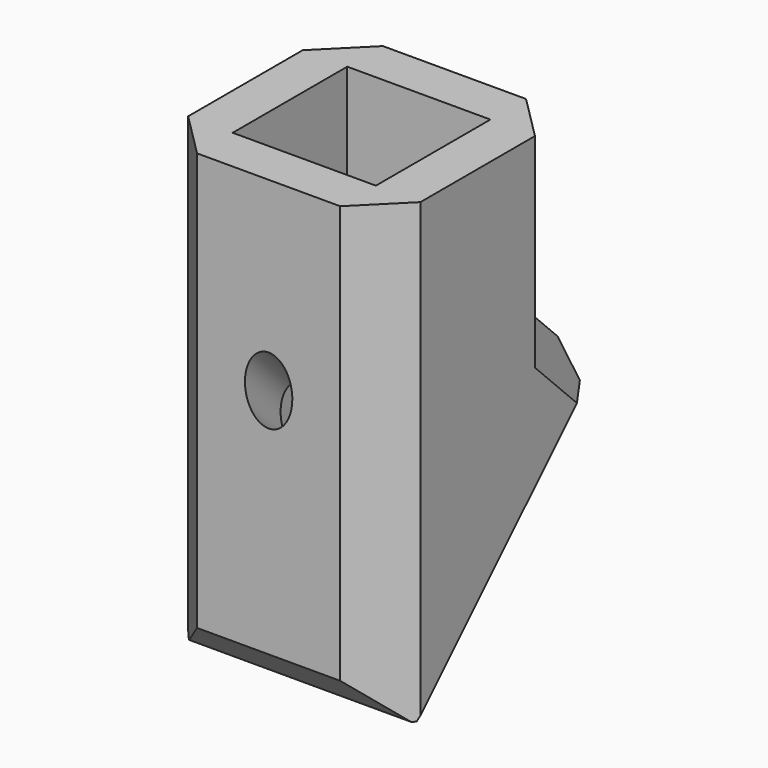
from build123d import *

# Parameters (mm, degrees)
F1_DEPTH    = 75
F3_DEPTH    = 41.701
F4_W        = 41.7
F4_H        = 58.972705551
F5_DEPTH    = 15
F6_R        = 11.05
F7_DEPTH    = 7
F8_R        = 4.25
F9_DEPTH    = 61.034008589
F10_SIZE    = 8
F12_C1_SIZE = 5
F12_C2_SIZE = 5
F12_C3_SIZE = 5
F12_C4_SIZE = 5
F13_SIZE    = 8


with BuildPart() as f1:
    # F0 (on Top) → F1 (new body)
    with BuildSketch(Plane.XY):
        Polygon((20.85, 20.85), (0, 20.85), (-20.85, 20.85), (-20.85, 0), (-20.85, -20.85), (0, -20.85), (20.85, -20.85), (20.85, 0), align=None)
        Polygon((-12.85, 12.85), (0, 12.85), (12.85, 12.85), (12.85, 0), (12.85, -12.85), (0, -12.85), (-12.85, -12.85), (-12.85, 0), align=None, mode=Mode.SUBTRACT)
    extrude(amount=F1_DEPTH)

    # F2 (on face) → F3 (cut, through all)
    with BuildSketch(Plane(origin=(-20.85, 0, 0), x_dir=(0, -1, 0), z_dir=(-1, 0, 0))):
        Polygon((-20.85, 0), (20.85, 0), (-20.85, 41.7), align=None)
    extrude(amount=-F3_DEPTH, mode=Mode.SUBTRACT)

    # F4 (on face) → F5 (join)
    with BuildSketch(Plane(origin=(0, -10.425, 10.425), x_dir=(1, 0, 0), z_dir=(0, 0.7071067812, -0.7071067812))):
        with Locations((0, -14.7431763877)):
            Rectangle(F4_W, F4_H)
    extrude(amount=F5_DEPTH)

    # F6 (on face) → F7 (cut)
    with BuildSketch(Plane(origin=(0, 0.1816017178, -0.1816017178), x_dir=(1, 0, 0), z_dir=(0, 0.7071067812, -0.7071067812))):
        with Locations((0, -14.7431763877)):
            Circle(F6_R)
    extrude(amount=-F7_DEPTH, mode=Mode.SUBTRACT)

    # F8 (on face) → F9 (cut, through all)
    with BuildSketch(Plane(origin=(0, -4.7681457505, 4.7681457505), x_dir=(1, 0, 0), z_dir=(0, 0.7071067812, -0.7071067812))):
        with Locations((0, -14.7431763877)):
            Circle(F8_R)
    extrude(amount=-F9_DEPTH, mode=Mode.SUBTRACT)

    # F10
    f10_edges = [f1.edges().sort_by_distance(p)[0] for p in [
        (-20.85, -20.85, 37.5),
        (20.85, -20.85, 37.5),
        (20.85, 20.85, 58.35),
        (-20.85, 20.85, 58.35),
    ]]
    chamfer(f10_edges, length=F10_SIZE)

    # F12: chamfer of 5 on 4 edges, made by hand

    # F12_c1
    f12_c1_edges = [f1.edges().sort_by_distance(p)[0] for p in [
        (0, 31.4566017178, 31.0933982822),
    ]]
    chamfer(f12_c1_edges, length=F12_C1_SIZE)

    # F12_c2
    f12_c2_edges = [f1.edges().sort_by_distance(p)[0] for p in [
        (-20.85, 8.8388347648, 8.4756313292),
    ]]
    chamfer(f12_c2_edges, length=F12_C2_SIZE)

    # F12_c3
    f12_c3_edges = [f1.edges().sort_by_distance(p)[0] for p in [
        (20.85, 8.8388347648, 8.4756313292),
    ]]
    chamfer(f12_c3_edges, length=F12_C3_SIZE)

    # F12_c4
    f12_c4_edges = [f1.edges().sort_by_distance(p)[0] for p in [
        (0, -10.2433982822, -10.6066017178),
    ]]
    chamfer(f12_c4_edges, length=F12_C4_SIZE)

    # F13
    f13_edges = [f1.edges().sort_by_distance(p)[0] for p in [
        (20.85, 24.385534, 38.164466),
        (-20.85, 24.385534, 38.164466),
    ]]
    chamfer(f13_edges, length=F13_SIZE)


solid = f1.part
